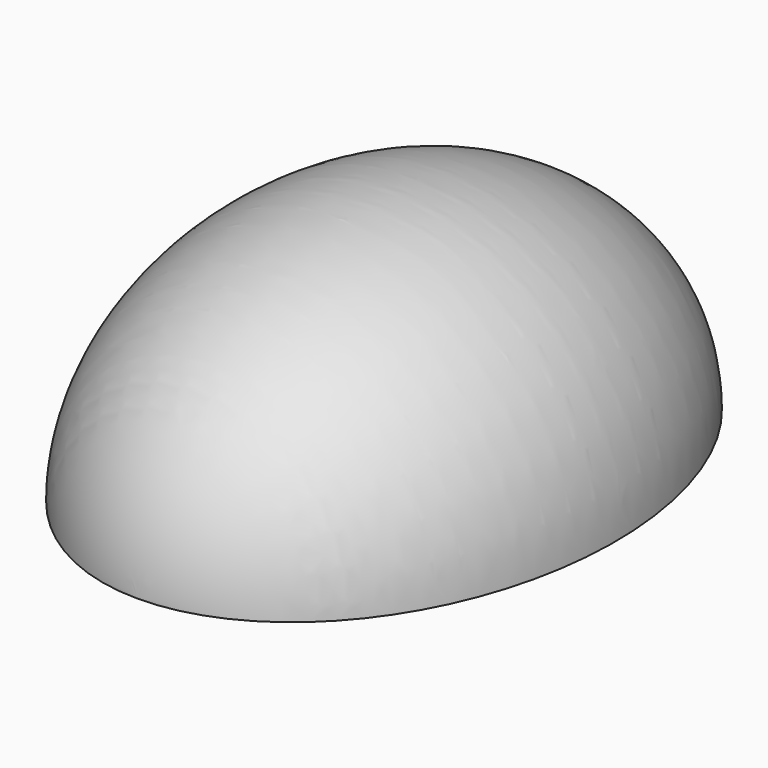
from build123d import *

# Parameters (mm, degrees)
F1_ANGLE = 180


# Not quite as in the source:
# - ends of sketch curves that miss each other by under 0.0002 mm in the source are joined


with BuildPart() as f1:
    # F0 (on Top) → F1 (revolve)
    with BuildSketch(Plane.XY):
        with BuildLine():
            Line((0, -40), (0, 40))
            add(Edge.make_bspline(
                [(0, 40), (-30.000001606, 39.999997591), (-30, -2.677e-07), (-29.999998394, -39.9999981263), (0, -40)],
                knots=[0, 0, 0, 1.5707962733, 1.5707962733, 3.1415925465, 3.1415925465, 3.1415925465], degree=2, weights=[1, 0.7071068001, 1, 0.7071068001, 1]))
        make_face()
    revolve(axis=Axis((0, 0, 0), (0, 1, 0)), revolution_arc=F1_ANGLE)


solid = f1.part
